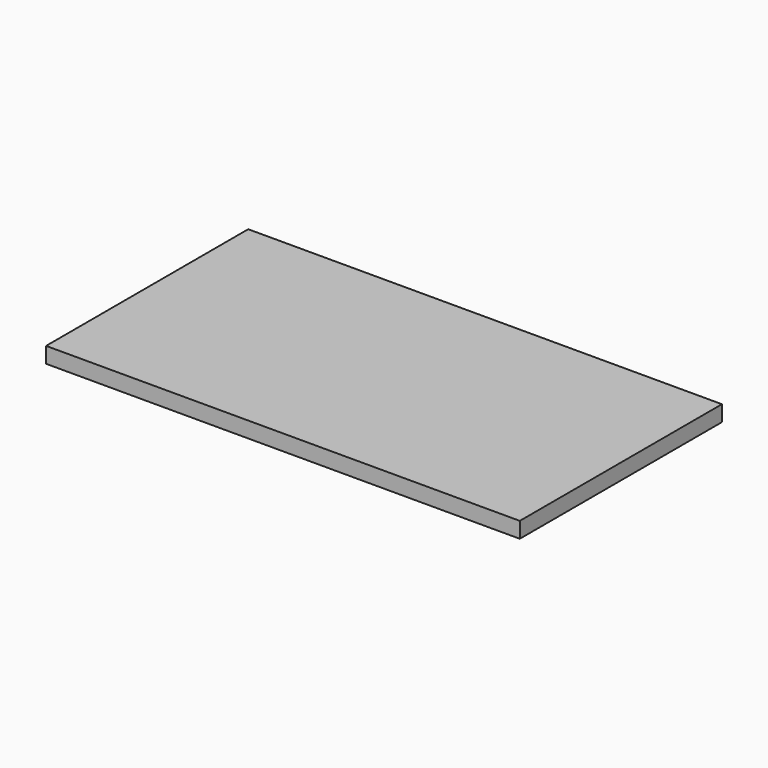
from build123d import *

# Parameters (mm, degrees)
F0_W     = 571.5
F0_H     = 304.8
F1_DEPTH = 19.05


# Not quite as in the source:
# - a feature names something its author has since deleted; it is built from what else it names


with BuildPart() as f1:
    # F0 (on Top) → F1 (new body)
    with BuildSketch(Plane.XY):
        Rectangle(F0_W, F0_H)
    extrude(amount=F1_DEPTH)


solid = f1.part
